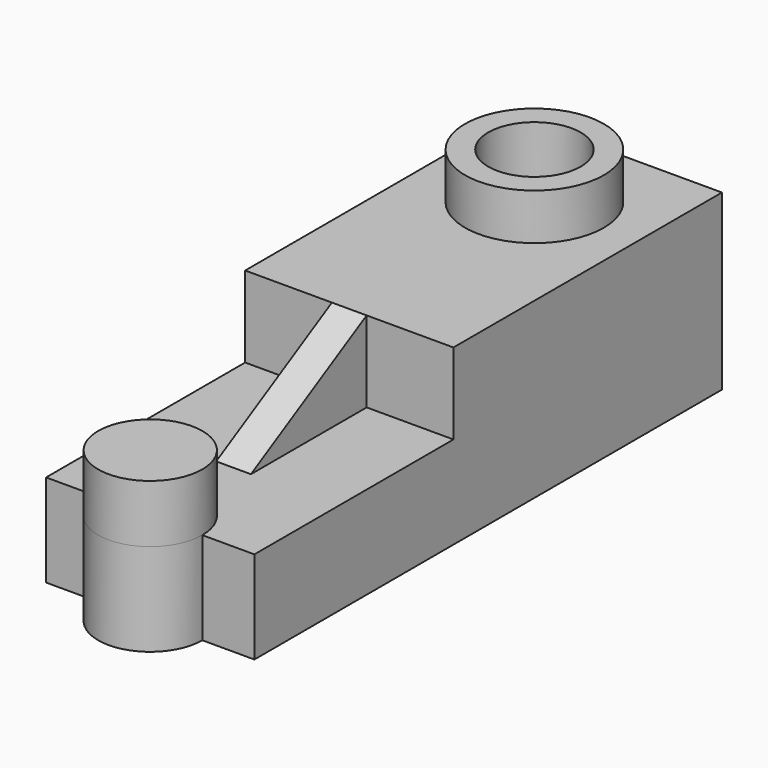
from build123d import *
from build123d import SkipClean  # not in build123d's __all__

# Parameters (mm, degrees)
F0_W      = 101
F0_H      = 30
F1_DEPTH  = 18
F2_R      = 12
F3_DEPTH  = 8
F4_R      = 8
F5_DEPTH  = 38.001
F6_W      = 43
F6_H      = 14
F7_DEPTH  = 36.001
F9_DEPTH  = 16
F8_R      = 9
F10_DEPTH = 10
F12_DEPTH = 3
F13_R     = 8
F14_DEPTH = 22
F16_DEPTH = 7


# Not quite as in the source:
# - after a boolean that leaves OpenCascade's solid faulty, fix() repairs it


with BuildPart() as f1:
    # F0 (on Right) → F1 (new body, symmetric)
    with BuildSketch(Plane.YZ):
        Rectangle(F0_W, F0_H)
    extrude(amount=F1_DEPTH, both=True)

    # F2 (on face) → F3 (join)
    with BuildSketch(Plane.XY.offset(15)):
        with Locations((0, 32.5)):
            Circle(F2_R)
    extrude(amount=F3_DEPTH)

    # F4 (on face) → F5 (cut, through all)
    with BuildSketch(Plane.XY.offset(23)):
        with Locations((0, 32.5)):
            Circle(F4_R)
    extrude(amount=-F5_DEPTH, mode=Mode.SUBTRACT)

    # F6 (on face) → F7 (cut, through all)
    with BuildSketch(Plane.YZ.offset(18)):
        with Locations((-29, 8)):
            Rectangle(F6_W, F6_H)
    extrude(amount=-F7_DEPTH, mode=Mode.SUBTRACT)

    # F8 (on face) → F9 (join)
    with BuildSketch(Plane.XY.offset(1)):
        with BuildLine():
            Line((-9, -50.5), (9, -50.5))
            ThreePointArc((9, -50.5), (0, -41.5), (-9, -50.5))
        make_face()
        with BuildLine():
            ThreePointArc((-9, -50.5), (0, -59.5), (9, -50.5))
            Line((9, -50.5), (-9, -50.5))
        make_face()
    extrude(amount=-F9_DEPTH)

    # F8 (on face) → F10 (join)
    with BuildSketch(Plane.XY.offset(1)):
        with Locations((0, -50.5)):
            Circle(F8_R)
    with SkipClean():  # cleaning this boolean's faces spoils the solid; the shape is the same uncleaned
        extrude(amount=F10_DEPTH)

    # F11 (on Right) → F12 (join, symmetric)
    with BuildSketch(Plane.YZ):
        Polygon((-7.5, 1), (-7.5, 15), (-32.5, 1), align=None)
    extrude(amount=F12_DEPTH, both=True)

    add(f1.part.fix(), mode=Mode.REPLACE)

    # F13 (on face) → F14 (cut)
    with BuildSketch(Plane(origin=(0, 0, -15), x_dir=(1, 0, 0), z_dir=(0, 0, -1))):
        with BuildLine():
            Line((-14, 2.5), (-14, -32.5))
            ThreePointArc((-14, -32.5), (0, -46.5), (14, -32.5))
            Line((14, -32.5), (14, 2.5))
            Line((14, 2.5), (-14, 2.5))
        make_face()
        with Locations((0, -32.5)):
            Circle(F13_R, mode=Mode.SUBTRACT)
    extrude(amount=-F14_DEPTH, mode=Mode.SUBTRACT)

    # F15 (on face) → F16 (cut)
    with BuildSketch(Plane(origin=(0, 0, -15), x_dir=(1, 0, 0), z_dir=(0, 0, -1))):
        with BuildLine():
            Line((9, 2.5), (9, 27.5))
            ThreePointArc((9, 27.5), (0, 36.5), (-9, 27.5))
            Line((-9, 27.5), (-9, 2.5))
            Line((-9, 2.5), (9, 2.5))
        make_face()
    extrude(amount=-F16_DEPTH, mode=Mode.SUBTRACT)


solid = f1.part
